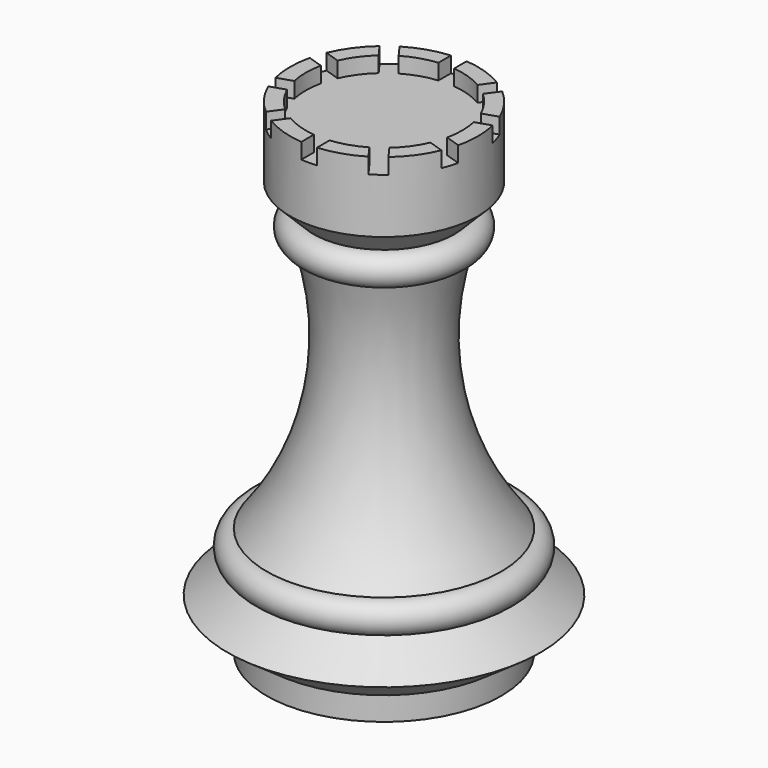
from build123d import *

# Parameters (mm, degrees)
F2_W            = 2.54
F2_H            = 2.54
F3_DEPTH        = 25.401
F3_DEPTH_BACK   = 25.401
F3_COPIES_COUNT = 5
F3_COPIES_ANGLE = 144


# Not quite as in the source:
# - a pattern or mirror of a feature is missing from the dataset's text; its kind, count and spacing are read off the source's solid


with BuildPart() as f1:
    # F0 (on Front) → F1 (revolve)
    with BuildSketch(Plane.XZ):
        with BuildLine():
            Line((0, 76.2), (0, 0))
            Line((0, 0), (19.05, 0))
            Line((19.05, 0), (19.05, 3.81))
            Line((19.05, 3.81), (25.4, 8.255))
            Line((25.4, 8.255), (19.05, 12.7))
            ThreePointArc((19.05, 12.7), (21.59, 15.24), (19.05, 17.78))
            ThreePointArc((19.05, 17.78), (10.2268710231, 37.1600383168), (11.43, 58.42))
            ThreePointArc((11.43, 58.42), (13.97, 60.96), (11.43, 63.5))
            Line((11.43, 63.5), (15.24, 67.31))
            Line((15.24, 67.31), (15.24, 78.74))
            Line((15.24, 78.74), (12.7, 78.74))
            Line((12.7, 78.74), (12.7, 76.2))
            Line((12.7, 76.2), (0, 76.2))
        make_face()
    revolve(axis=Axis((0, 0, 38.1), (0, 0, 1)))

    # F2 (on Front) → F3 (cut, two sides)
    with BuildSketch(Plane.XZ) as f3_sk:
        with Locations((0, 77.47)):
            Rectangle(F2_W, F2_H)
    f3 = extrude(amount=-F3_DEPTH, mode=Mode.SUBTRACT) + extrude(f3_sk.sketch, amount=F3_DEPTH_BACK, mode=Mode.SUBTRACT)

    # F3_copies: F3 ×5 about axis
    f3_copies_axis = Axis((0, 0, 0), (0, 0, 1))
    for i in range(1, F3_COPIES_COUNT):
        add(f3.rotate(f3_copies_axis, i * F3_COPIES_ANGLE / (F3_COPIES_COUNT - 1)), mode=Mode.SUBTRACT)


solid = f1.part
